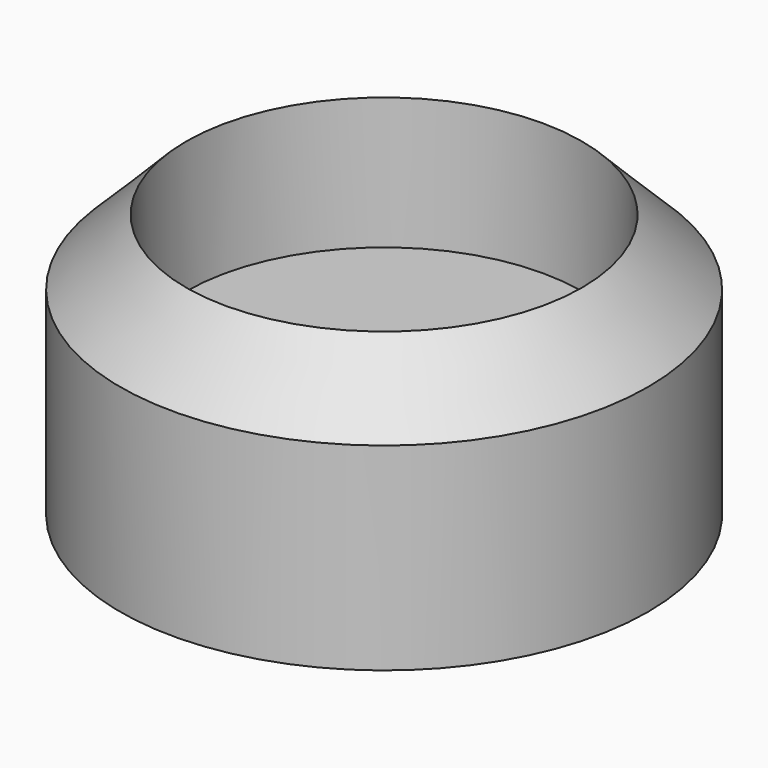
from build123d import *

# Parameters (mm, degrees)
F0_R     = 50.8
F1_DEPTH = 50.8
F2_SIZE  = 12.7
F3_DEPTH = 25.4
F4_T     = 6.35


# Not quite as in the source:
# - a shell that OpenCascade refuses in one call is made with other operations: the cavity is built on its own and cut out


with BuildPart() as f1:
    # F0 (on Top) → F1 (new body)
    with BuildSketch(Plane.XY):
        Circle(F0_R)
    extrude(amount=F1_DEPTH)

    # F2
    f2_edges = [f1.edges().sort_by_distance(p)[0] for p in [
        (-50.8, 0, 50.8),
    ]]
    chamfer(f2_edges, length=F2_SIZE)

    # F3 (cut): a face of the model
    f3_faces = [f1.faces().sort_by_distance(p)[0] for p in [
        (0, 0, 50.8),
    ]]
    extrude(f3_faces, amount=-F3_DEPTH, mode=Mode.SUBTRACT)

    # F4: shell of thickness 6.35, made by hand


with BuildPart() as f4_core1:
    # F4_t2: copy of F1
    add(f1.part)

    # the walls: a layer under each face that stays
    f4_faces = [f4_core1.faces().sort_by_distance(p)[0] for p in [
        (-50.8, 0, 19.05),
        (-44.45, 0, 44.45),
        (-38.1, 0, 38.1),
        (0, 0, 25.4),
    ]]
    thicken(f4_faces, amount=-F4_T, mode=Mode.SUBTRACT)

    # F4_s3 → F4_t4 (revolve, cut)
    with BuildSketch(Plane.XZ):
        Polygon((38.0365, 25.4635), (44.45, 25.4), (44.45, 19.05), (38.1, 19.05), align=None)
    revolve(axis=Axis((0, 0, 25.4), (0, 0, 1)), mode=Mode.SUBTRACT)


with BuildPart() as f1_1:
    add(f1.part)

    # what is left inside the walls is the cavity
    f4_cavity = [f4_core1.part.solids().sort_by_distance(p)[0] for p in [
        (0, -14.816667, 18.9865),
    ]]
    add(f4_cavity, mode=Mode.SUBTRACT)


solid = f1_1.part
